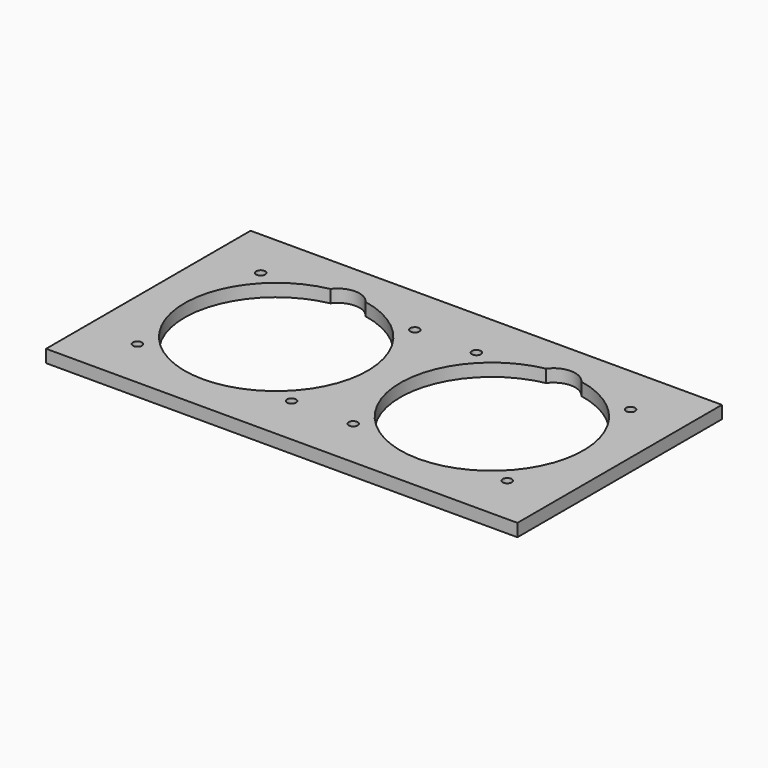
from build123d import *

# Parameters (mm, degrees)
F0_W     = 130
F0_H     = 70.5
F1_DEPTH = 3.5
F2_D     = 2.5


# Not quite as in the source:
# - a feature names something its author has since deleted; it is built from what else it names


with BuildPart() as f1:
    # F0 (on Top) → F1 (new body)
    with BuildSketch(Plane.XY):
        Rectangle(F0_W, F0_H)
        with BuildLine():
            ThreePointArc((-24.8978610289, 24.7794117647), (-29.75, -25.25), (-34.6021389711, 24.7794117647))
            ThreePointArc((-34.6021389711, 24.7794117647), (-29.75, 27.25), (-24.8978610289, 24.7794117647))
        make_face(mode=Mode.SUBTRACT)
        with BuildLine():
            ThreePointArc((34.6021389711, 24.7794117647), (29.75, -25.25), (24.8978610289, 24.7794117647))
            ThreePointArc((24.8978610289, 24.7794117647), (29.75, 27.25), (34.6021389711, 24.7794117647))
        make_face(mode=Mode.SUBTRACT)
    extrude(amount=F1_DEPTH)

    # F2 (through all)
    with Locations(Plane(origin=(0, 0, 0), x_dir=(1, 0, 0), z_dir=(0, 0, -1))):
        with Locations((-51, -21.25), (-51, 21.25), (-8.5, 21.25), (-8.5, -21.25), (8.5, -21.25), (8.5, 21.25), (51, 21.25), (51, -21.25)):
            Hole(F2_D / 2)


solid = f1.part
